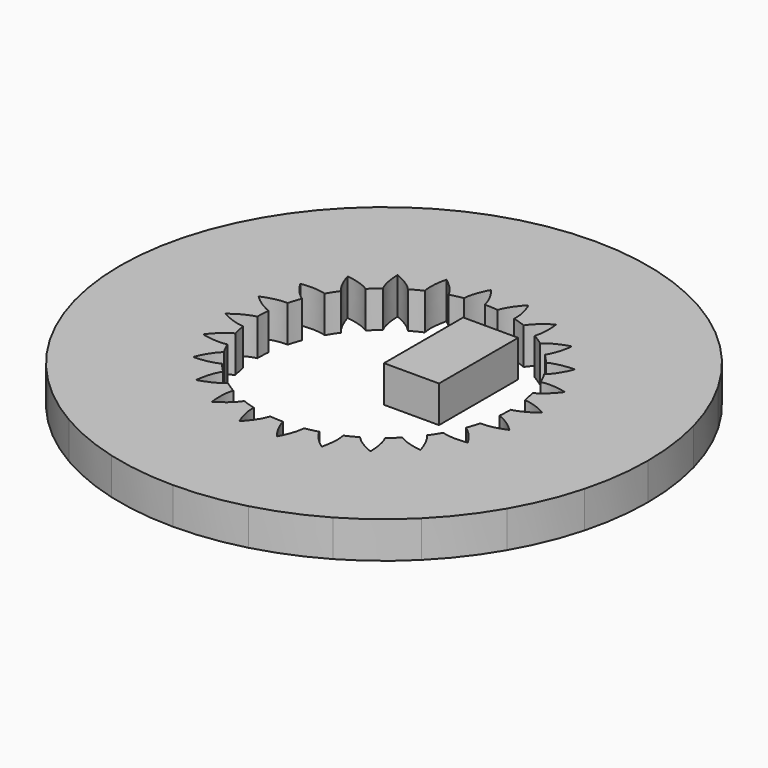
from build123d import *

# Parameters (mm, degrees)
F4_DEPTH = 10
F6_COUNT = 24
F7_W     = 15
F7_H     = 27
F8_DEPTH = 10


# Not quite as in the source:
# - the dataset's text gives a spline's control points without its knots; the knots are read off the source's solid
# - a feature names something its author has since deleted; it is built from what else it names


with BuildPart() as f4:
    # F3 (on Top) → F4 (new body)
    with BuildSketch(Plane.XY):
        with BuildLine():
            Line((-18.6349712474, 69.5466594928), (-10.6762856105, 39.8444403344))
            ThreePointArc((-10.6762856105, 39.8444403344), (-7.1888090971, 40.6187582745), (-3.6474150708, 41.0884273647))
            ThreePointArc((-3.6474150708, 41.0884273647), (-3.3110461109, 41.1169000978), (-2.9744554081, 41.1426192047))
            add(Edge.make_bspline(
                [(-2.9744554081, 41.1426192047), (-2.9729446939, 41.1451563137), (-2.7929354809, 41.44733642), (-2.4095701, 42.059784773), (-1.7708367652, 42.9879740234), (-1.0509773523, 43.9409278123), (-0.4523761322, 44.667921636), (-0.0839892413, 45.0876480338), (0, 45.1822032449)],
                knots=[0.5442094806, 0.5442094806, 0.5442094806, 0.5442094806, 0.5446479585, 0.5964327949, 0.6497637866, 0.7045973538, 0.7608934059, 0.7773380693, 0.7773380693, 0.7773380693, 0.7773380693], degree=3))
            Line((0, 45.1822032449), (0, 72))
            ThreePointArc((0, 72), (-9.3978858398, 71.3840300189), (-18.6349712474, 69.5466594928))
        make_face()
        with BuildLine():
            ThreePointArc((-2.9744554081, 41.1426192047), (-1.4881965268, 41.2231460602), (0, 41.25))
            Line((0, 41.25), (0, 45.1822032449))
            add(Edge.make_bspline(
                [(-2.9744554081, 41.1426192047), (-2.9729446939, 41.1451563137), (-2.7929354809, 41.44733642), (-2.4095701, 42.059784773), (-1.7708367652, 42.9879740234), (-1.0509773523, 43.9409278123), (-0.4523761322, 44.667921636), (-0.0839892413, 45.0876480338), (0, 45.1822032449)],
                knots=[0.5442094806, 0.5442094806, 0.5442094806, 0.5442094806, 0.5446479585, 0.5964327949, 0.6497637866, 0.7045973538, 0.7608934059, 0.7773380693, 0.7773380693, 0.7773380693, 0.7773380693], degree=3))
        make_face()
        with BuildLine():
            ThreePointArc((-0.0900286505, 34.4998825337), (-0.0450143636, 34.4999706334), (0, 34.5))
            Line((0, 34.5), (0, 41.25))
            ThreePointArc((0, 41.25), (-1.4881965268, 41.2231460602), (-2.9744554081, 41.1426192047))
            add(Edge.make_bspline(
                [(-3.2717235535, 40.6285887043), (-3.1757650344, 40.7995707867), (-3.0766694054, 40.9709599615), (-2.9744554081, 41.1426192047)],
                knots=[0.5145423288, 0.5145423288, 0.5145423288, 0.5145423288, 0.5442094806, 0.5442094806, 0.5442094806, 0.5442094806], degree=3))
            add(Edge.make_bspline(
                [(-0.0900286505, 34.4998825337), (-0.0982987917, 34.5405905939), (-0.1300142008, 34.6896241293), (-0.1996473151, 34.9745158078), (-0.3168142765, 35.3763667744), (-0.4721193842, 35.8339154879), (-0.6705802963, 36.3442430463), (-0.9170594192, 36.9044110793), (-1.2162308733, 37.5110684286), (-1.5725655088, 38.160580156), (-1.9903130634, 38.8490053284), (-2.4734792066, 39.5721160186), (-2.9116042188, 40.1696372334), (-3.1890707253, 40.524716757), (-3.2717235612, 40.628588706)],
                knots=[0.0841349721, 0.0841349721, 0.0841349721, 0.0841349721, 0.0956797746, 0.1255777668, 0.1580803099, 0.1929936411, 0.2301617199, 0.2694553768, 0.3107653862, 0.3539978077, 0.3990707228, 0.44591187, 0.4944568849, 0.5145423289, 0.5145423289, 0.5145423289, 0.5145423289], degree=3))
        make_face()
        with BuildLine():
            Line((-10.6762856105, 39.8444403344), (-8.929257056, 33.324441007))
            ThreePointArc((-8.929257056, 33.324441007), (-7.1901510163, 33.7424321643), (-5.4317189717, 34.0697289248))
            add(Edge.make_bspline(
                [(-5.4317189717, 34.0697289248), (-5.4300694033, 34.1112357956), (-5.4226106586, 34.2634239324), (-5.3994625004, 34.5557870659), (-5.3481085501, 34.9712086205), (-5.2680205137, 35.4477129837), (-5.1537783143, 35.9832217795), (-5.0001120106, 36.5756125713), (-4.8018714679, 37.2223253249), (-4.5540617929, 37.9204873558), (-4.2518573905, 38.666888546), (-3.8906276651, 39.4579964259), (-3.5537621552, 40.1179257823), (-3.3366900009, 40.5128293265), (-3.2717235535, 40.6285887043)],
                knots=[0.0841349721, 0.0841349721, 0.0841349721, 0.0841349721, 0.0956797746, 0.1255777668, 0.1580803099, 0.1929936411, 0.2301617199, 0.2694553768, 0.3107653862, 0.3539978077, 0.3990707228, 0.44591187, 0.4944568849, 0.5145423288, 0.5145423288, 0.5145423288, 0.5145423288], degree=3))
            add(Edge.make_bspline(
                [(-3.2717235612, 40.628588706), (-3.3938057124, 40.7820124914), (-3.519049691, 40.9353361307), (-3.6474150708, 41.0884273647)],
                knots=[0.5145423289, 0.5145423289, 0.5145423289, 0.5145423289, 0.5442094806, 0.5442094806, 0.5442094806, 0.5442094806], degree=3))
            ThreePointArc((-3.6474150708, 41.0884273647), (-7.1888090971, 40.6187582745), (-10.6762856105, 39.8444403344))
        make_face()
        with BuildLine():
            add(Edge.make_bspline(
                [(-3.2717235612, 40.628588706), (-3.3938057124, 40.7820124914), (-3.519049691, 40.9353361307), (-3.6474150708, 41.0884273647)],
                knots=[0.5145423289, 0.5145423289, 0.5145423289, 0.5145423289, 0.5442094806, 0.5442094806, 0.5442094806, 0.5442094806], degree=3))
            add(Edge.make_bspline(
                [(-3.2717235535, 40.6285887043), (-3.1757650344, 40.7995707867), (-3.0766694054, 40.9709599615), (-2.9744554081, 41.1426192047)],
                knots=[0.5145423288, 0.5145423288, 0.5145423288, 0.5145423288, 0.5442094806, 0.5442094806, 0.5442094806, 0.5442094806], degree=3))
            ThreePointArc((-2.9744554081, 41.1426192047), (-3.3110461109, 41.1169000978), (-3.6474150708, 41.0884273647))
        make_face()
    extrude(amount=F4_DEPTH)

    # F6: F4 ×24 about axis
    f6_axis = Axis((0, 0, 19.9973106452), (0, 0, 1))


with BuildPart() as f4_1:
    add(f4.part)
    for i in range(1, F6_COUNT):
        add(f4.part.rotate(f6_axis, i * 360 / F6_COUNT))


with BuildPart() as f8:
    # F7 (on Top) → F8 (new body)
    with BuildSketch(Plane.XY):
        with Locations((7.5, 13.5)):
            Rectangle(F7_W, F7_H)
    extrude(amount=F8_DEPTH)


solid = Compound([f4_1.part, f8.part])
